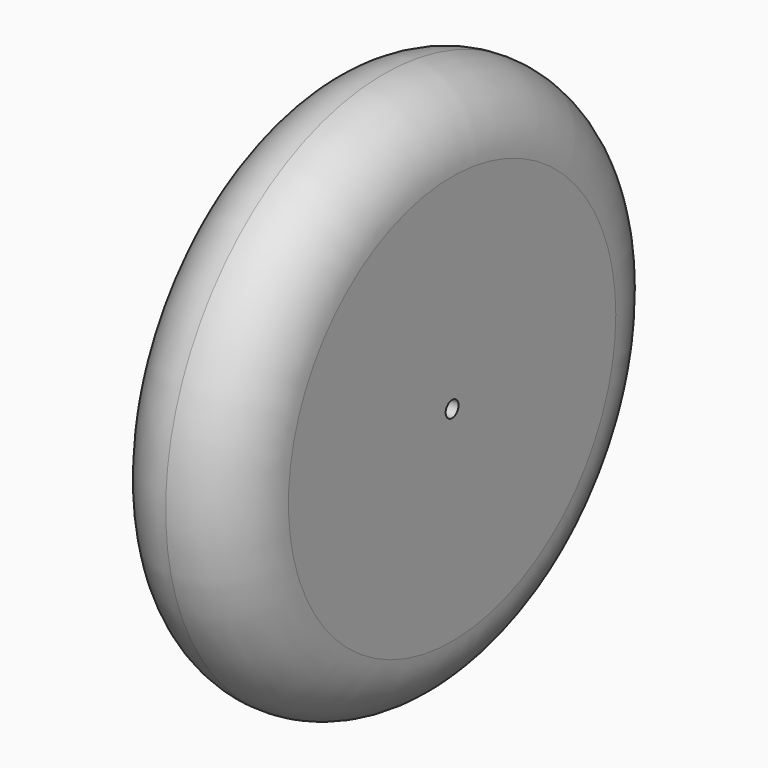
from build123d import *

# Parameters (mm, degrees)
F0_R     = 50.8
F1_DEPTH = 25.4
F2_R     = 12.7
F3_R     = 12.69999
F5_D     = 2.999994


# Not quite as in the source:
# - a fillet or chamfer is up to 0.001 mm smaller than in the source, because OpenCascade refuses the exact size


with BuildPart() as f1:
    # F0 (on Right) → F1 (new body)
    with BuildSketch(Plane.YZ):
        Circle(F0_R)
    extrude(amount=F1_DEPTH)

    # F2
    f2_edges = [f1.edges().sort_by_distance(p)[0] for p in [
        (25.4, -50.8, 0),
    ]]
    fillet(f2_edges, radius=F2_R)

    # F3 (radius 12.7 in the source; OpenCascade refuses exactly that, so slightly less here)
    f3_edges = [f1.edges().sort_by_distance(p)[0] for p in [
        (0, -50.8, 0),
    ]]
    fillet(f3_edges, radius=F3_R)

    # F5 (through all)
    with Locations(Plane.YZ.offset(25.4)):
        with Locations((0, 0)):
            Hole(F5_D / 2)


solid = f1.part
